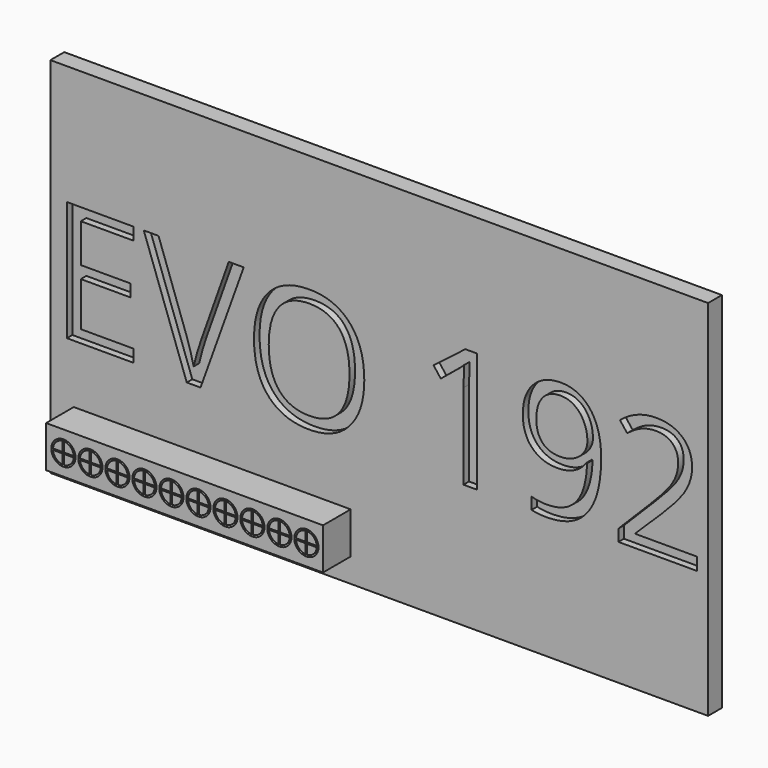
from build123d import *

# Parameters (mm, degrees)
F0_W         = 190
F0_H         = 105
F1_DEPTH     = 5
F2_TEXT_SIZE = 48.5157995531
F3_DEPTH     = 2
F4_W         = 80
F4_H         = 12
F4_R         = 3.5
F5_DEPTH     = 10


# Not quite as in the source:
# - Text() gives the source's letters only with a copy of the font that has no kerning and outlines rounded to 1/6400 em; it was checked with that copy


with BuildPart() as f1:
    # F0 (on Front) → F1 (new body)
    with BuildSketch(Plane.XZ):
        Rectangle(F0_W, F0_H)
    extrude(amount=F1_DEPTH)

    # F2 (on face) → F3 (cut)
    with BuildSketch(Plane.XZ.offset(5)):
        with Locations((-95, -16.6787064434)):
            Text('EVO 192', F2_TEXT_SIZE, font='Open Sans', text_align=(TextAlign.LEFT, TextAlign.BOTTOM))
    extrude(amount=-F3_DEPTH, mode=Mode.SUBTRACT)

    # F4 (on face) → F5 (join)
    with BuildSketch(Plane.XZ.offset(5)):
        with Locations((-48.2472097501, -39.5428631023)):
            Rectangle(F4_W, F4_H)
        with Locations((-83.2472097501, -39.5428631023)):
            Circle(F4_R, mode=Mode.SUBTRACT)
        with Locations((-75.4472097501, -39.5428631023)):
            Circle(F4_R, mode=Mode.SUBTRACT)
        with Locations((-67.6472097501, -39.5428631023)):
            Circle(F4_R, mode=Mode.SUBTRACT)
        with Locations((-59.8472097501, -39.5428631023)):
            Circle(F4_R, mode=Mode.SUBTRACT)
        with Locations((-52.0472097501, -39.5428631023)):
            Circle(F4_R, mode=Mode.SUBTRACT)
        with Locations((-44.2472097501, -39.5428631023)):
            Circle(F4_R, mode=Mode.SUBTRACT)
        with Locations((-36.4472097501, -39.5428631023)):
            Circle(F4_R, mode=Mode.SUBTRACT)
        with Locations((-28.6472097501, -39.5428631023)):
            Circle(F4_R, mode=Mode.SUBTRACT)
        with Locations((-20.8472097501, -39.5428631023)):
            Circle(F4_R, mode=Mode.SUBTRACT)
        with Locations((-13.0472097501, -39.5428631023)):
            Circle(F4_R, mode=Mode.SUBTRACT)
        with BuildLine():
            Line((-83.4472097501, -39.3428631023), (-83.4472097501, -36.5495371929))
            ThreePointArc((-83.4472097501, -36.5495371929), (-85.3685300937, -37.4215427588), (-86.2405356595, -39.3428631023))
            Line((-86.2405356595, -39.3428631023), (-83.4472097501, -39.3428631023))
        make_face()
        with BuildLine():
            Line((-83.0472097501, -39.3428631023), (-80.2538838407, -39.3428631023))
            ThreePointArc((-80.2538838407, -39.3428631023), (-81.1258894066, -37.4215427588), (-83.0472097501, -36.5495371929))
            Line((-83.0472097501, -36.5495371929), (-83.0472097501, -39.3428631023))
        make_face()
        with BuildLine():
            ThreePointArc((-83.0472097501, -42.5361890118), (-81.1258894066, -41.6641834459), (-80.2538838407, -39.7428631023))
            Line((-80.2538838407, -39.7428631023), (-83.0472097501, -39.7428631023))
            Line((-83.0472097501, -39.7428631023), (-83.0472097501, -42.5361890118))
        make_face()
        with BuildLine():
            ThreePointArc((-86.2405356595, -39.7428631023), (-85.3685300937, -41.6641834459), (-83.4472097501, -42.5361890118))
            Line((-83.4472097501, -42.5361890118), (-83.4472097501, -39.7428631023))
            Line((-83.4472097501, -39.7428631023), (-86.2405356595, -39.7428631023))
        make_face()
        with BuildLine():
            Line((-75.6472097501, -39.3428631023), (-75.6472097501, -36.5495371929))
            ThreePointArc((-75.6472097501, -36.5495371929), (-77.5685300937, -37.4215427588), (-78.4405356595, -39.3428631023))
            Line((-78.4405356595, -39.3428631023), (-75.6472097501, -39.3428631023))
        make_face()
        with BuildLine():
            Line((-75.2472097501, -39.3428631023), (-72.4538838407, -39.3428631023))
            ThreePointArc((-72.4538838407, -39.3428631023), (-73.3258894066, -37.4215427588), (-75.2472097501, -36.5495371929))
            Line((-75.2472097501, -36.5495371929), (-75.2472097501, -39.3428631023))
        make_face()
        with BuildLine():
            ThreePointArc((-75.2472097501, -42.5361890118), (-73.3258894066, -41.6641834459), (-72.4538838407, -39.7428631023))
            Line((-72.4538838407, -39.7428631023), (-75.2472097501, -39.7428631023))
            Line((-75.2472097501, -39.7428631023), (-75.2472097501, -42.5361890118))
        make_face()
        with BuildLine():
            ThreePointArc((-78.4405356595, -39.7428631023), (-77.5685300937, -41.6641834459), (-75.6472097501, -42.5361890118))
            Line((-75.6472097501, -42.5361890118), (-75.6472097501, -39.7428631023))
            Line((-75.6472097501, -39.7428631023), (-78.4405356595, -39.7428631023))
        make_face()
        with BuildLine():
            Line((-67.8472097501, -39.3428631023), (-67.8472097501, -36.5495371929))
            ThreePointArc((-67.8472097501, -36.5495371929), (-69.7685300937, -37.4215427588), (-70.6405356595, -39.3428631023))
            Line((-70.6405356595, -39.3428631023), (-67.8472097501, -39.3428631023))
        make_face()
        with BuildLine():
            Line((-67.4472097501, -39.3428631023), (-64.6538838407, -39.3428631023))
            ThreePointArc((-64.6538838407, -39.3428631023), (-65.5258894066, -37.4215427588), (-67.4472097501, -36.5495371929))
            Line((-67.4472097501, -36.5495371929), (-67.4472097501, -39.3428631023))
        make_face()
        with BuildLine():
            ThreePointArc((-67.4472097501, -42.5361890118), (-65.5258894066, -41.6641834459), (-64.6538838407, -39.7428631023))
            Line((-64.6538838407, -39.7428631023), (-67.4472097501, -39.7428631023))
            Line((-67.4472097501, -39.7428631023), (-67.4472097501, -42.5361890118))
        make_face()
        with BuildLine():
            ThreePointArc((-70.6405356595, -39.7428631023), (-69.7685300937, -41.6641834459), (-67.8472097501, -42.5361890118))
            Line((-67.8472097501, -42.5361890118), (-67.8472097501, -39.7428631023))
            Line((-67.8472097501, -39.7428631023), (-70.6405356595, -39.7428631023))
        make_face()
        with BuildLine():
            Line((-60.0472097501, -39.3428631023), (-60.0472097501, -36.5495371929))
            ThreePointArc((-60.0472097501, -36.5495371929), (-61.9685300937, -37.4215427588), (-62.8405356595, -39.3428631023))
            Line((-62.8405356595, -39.3428631023), (-60.0472097501, -39.3428631023))
        make_face()
        with BuildLine():
            Line((-59.6472097501, -39.3428631023), (-56.8538838407, -39.3428631023))
            ThreePointArc((-56.8538838407, -39.3428631023), (-57.7258894066, -37.4215427588), (-59.6472097501, -36.5495371929))
            Line((-59.6472097501, -36.5495371929), (-59.6472097501, -39.3428631023))
        make_face()
        with BuildLine():
            ThreePointArc((-59.6472097501, -42.5361890118), (-57.7258894066, -41.6641834459), (-56.8538838407, -39.7428631023))
            Line((-56.8538838407, -39.7428631023), (-59.6472097501, -39.7428631023))
            Line((-59.6472097501, -39.7428631023), (-59.6472097501, -42.5361890118))
        make_face()
        with BuildLine():
            ThreePointArc((-62.8405356595, -39.7428631023), (-61.9685300937, -41.6641834459), (-60.0472097501, -42.5361890118))
            Line((-60.0472097501, -42.5361890118), (-60.0472097501, -39.7428631023))
            Line((-60.0472097501, -39.7428631023), (-62.8405356595, -39.7428631023))
        make_face()
        with BuildLine():
            Line((-52.2472097501, -39.3428631023), (-52.2472097501, -36.5495371929))
            ThreePointArc((-52.2472097501, -36.5495371929), (-54.1685300937, -37.4215427588), (-55.0405356595, -39.3428631023))
            Line((-55.0405356595, -39.3428631023), (-52.2472097501, -39.3428631023))
        make_face()
        with BuildLine():
            Line((-51.8472097501, -39.3428631023), (-49.0538838407, -39.3428631023))
            ThreePointArc((-49.0538838407, -39.3428631023), (-49.9258894066, -37.4215427588), (-51.8472097501, -36.5495371929))
            Line((-51.8472097501, -36.5495371929), (-51.8472097501, -39.3428631023))
        make_face()
        with BuildLine():
            ThreePointArc((-51.8472097501, -42.5361890118), (-49.9258894066, -41.6641834459), (-49.0538838407, -39.7428631023))
            Line((-49.0538838407, -39.7428631023), (-51.8472097501, -39.7428631023))
            Line((-51.8472097501, -39.7428631023), (-51.8472097501, -42.5361890118))
        make_face()
        with BuildLine():
            ThreePointArc((-55.0405356595, -39.7428631023), (-54.1685300937, -41.6641834459), (-52.2472097501, -42.5361890118))
            Line((-52.2472097501, -42.5361890118), (-52.2472097501, -39.7428631023))
            Line((-52.2472097501, -39.7428631023), (-55.0405356595, -39.7428631023))
        make_face()
        with BuildLine():
            Line((-44.4472097501, -39.3428631023), (-44.4472097501, -36.5495371929))
            ThreePointArc((-44.4472097501, -36.5495371929), (-46.3685300937, -37.4215427588), (-47.2405356595, -39.3428631023))
            Line((-47.2405356595, -39.3428631023), (-44.4472097501, -39.3428631023))
        make_face()
        with BuildLine():
            Line((-44.0472097501, -39.3428631023), (-41.2538838407, -39.3428631023))
            ThreePointArc((-41.2538838407, -39.3428631023), (-42.1258894066, -37.4215427588), (-44.0472097501, -36.5495371929))
            Line((-44.0472097501, -36.5495371929), (-44.0472097501, -39.3428631023))
        make_face()
        with BuildLine():
            ThreePointArc((-44.0472097501, -42.5361890118), (-42.1258894066, -41.6641834459), (-41.2538838407, -39.7428631023))
            Line((-41.2538838407, -39.7428631023), (-44.0472097501, -39.7428631023))
            Line((-44.0472097501, -39.7428631023), (-44.0472097501, -42.5361890118))
        make_face()
        with BuildLine():
            ThreePointArc((-47.2405356595, -39.7428631023), (-46.3685300937, -41.6641834459), (-44.4472097501, -42.5361890118))
            Line((-44.4472097501, -42.5361890118), (-44.4472097501, -39.7428631023))
            Line((-44.4472097501, -39.7428631023), (-47.2405356595, -39.7428631023))
        make_face()
        with BuildLine():
            Line((-36.2472097501, -39.3428631023), (-33.4538838407, -39.3428631023))
            ThreePointArc((-33.4538838407, -39.3428631023), (-34.3258894066, -37.4215427588), (-36.2472097501, -36.5495371929))
            Line((-36.2472097501, -36.5495371929), (-36.2472097501, -39.3428631023))
        make_face()
        with BuildLine():
            Line((-36.6472097501, -39.3428631023), (-36.6472097501, -36.5495371929))
            ThreePointArc((-36.6472097501, -36.5495371929), (-38.5685300937, -37.4215427588), (-39.4405356595, -39.3428631023))
            Line((-39.4405356595, -39.3428631023), (-36.6472097501, -39.3428631023))
        make_face()
        with BuildLine():
            ThreePointArc((-39.4405356595, -39.7428631023), (-38.5685300937, -41.6641834459), (-36.6472097501, -42.5361890118))
            Line((-36.6472097501, -42.5361890118), (-36.6472097501, -39.7428631023))
            Line((-36.6472097501, -39.7428631023), (-39.4405356595, -39.7428631023))
        make_face()
        with BuildLine():
            ThreePointArc((-36.2472097501, -42.5361890118), (-34.3258894066, -41.6641834459), (-33.4538838407, -39.7428631023))
            Line((-33.4538838407, -39.7428631023), (-36.2472097501, -39.7428631023))
            Line((-36.2472097501, -39.7428631023), (-36.2472097501, -42.5361890118))
        make_face()
        with BuildLine():
            Line((-28.8472097501, -39.3428631023), (-28.8472097501, -36.5495371929))
            ThreePointArc((-28.8472097501, -36.5495371929), (-30.7685300937, -37.4215427588), (-31.6405356595, -39.3428631023))
            Line((-31.6405356595, -39.3428631023), (-28.8472097501, -39.3428631023))
        make_face()
        with BuildLine():
            Line((-28.4472097501, -39.3428631023), (-25.6538838407, -39.3428631023))
            ThreePointArc((-25.6538838407, -39.3428631023), (-26.5258894066, -37.4215427588), (-28.4472097501, -36.5495371929))
            Line((-28.4472097501, -36.5495371929), (-28.4472097501, -39.3428631023))
        make_face()
        with BuildLine():
            ThreePointArc((-28.4472097501, -42.5361890118), (-26.5258894066, -41.6641834459), (-25.6538838407, -39.7428631023))
            Line((-25.6538838407, -39.7428631023), (-28.4472097501, -39.7428631023))
            Line((-28.4472097501, -39.7428631023), (-28.4472097501, -42.5361890118))
        make_face()
        with BuildLine():
            ThreePointArc((-31.6405356595, -39.7428631023), (-30.7685300937, -41.6641834459), (-28.8472097501, -42.5361890118))
            Line((-28.8472097501, -42.5361890118), (-28.8472097501, -39.7428631023))
            Line((-28.8472097501, -39.7428631023), (-31.6405356595, -39.7428631023))
        make_face()
        with BuildLine():
            Line((-21.0472097501, -39.3428631023), (-21.0472097501, -36.5495371929))
            ThreePointArc((-21.0472097501, -36.5495371929), (-22.9685300937, -37.4215427588), (-23.8405356595, -39.3428631023))
            Line((-23.8405356595, -39.3428631023), (-21.0472097501, -39.3428631023))
        make_face()
        with BuildLine():
            Line((-20.6472097501, -39.3428631023), (-17.8538838407, -39.3428631023))
            ThreePointArc((-17.8538838407, -39.3428631023), (-18.7258894066, -37.4215427588), (-20.6472097501, -36.5495371929))
            Line((-20.6472097501, -36.5495371929), (-20.6472097501, -39.3428631023))
        make_face()
        with BuildLine():
            ThreePointArc((-20.6472097501, -42.5361890118), (-18.7258894066, -41.6641834459), (-17.8538838407, -39.7428631023))
            Line((-17.8538838407, -39.7428631023), (-20.6472097501, -39.7428631023))
            Line((-20.6472097501, -39.7428631023), (-20.6472097501, -42.5361890118))
        make_face()
        with BuildLine():
            ThreePointArc((-23.8405356595, -39.7428631023), (-22.9685300937, -41.6641834459), (-21.0472097501, -42.5361890118))
            Line((-21.0472097501, -42.5361890118), (-21.0472097501, -39.7428631023))
            Line((-21.0472097501, -39.7428631023), (-23.8405356595, -39.7428631023))
        make_face()
        with BuildLine():
            Line((-13.2472097501, -39.3428631023), (-13.2472097501, -36.5495371929))
            ThreePointArc((-13.2472097501, -36.5495371929), (-15.1685300937, -37.4215427588), (-16.0405356595, -39.3428631023))
            Line((-16.0405356595, -39.3428631023), (-13.2472097501, -39.3428631023))
        make_face()
        with BuildLine():
            Line((-12.8472097501, -39.3428631023), (-10.0538838407, -39.3428631023))
            ThreePointArc((-10.0538838407, -39.3428631023), (-10.9258894066, -37.4215427588), (-12.8472097501, -36.5495371929))
            Line((-12.8472097501, -36.5495371929), (-12.8472097501, -39.3428631023))
        make_face()
        with BuildLine():
            ThreePointArc((-12.8472097501, -42.5361890118), (-10.9258894066, -41.6641834459), (-10.0538838407, -39.7428631023))
            Line((-10.0538838407, -39.7428631023), (-12.8472097501, -39.7428631023))
            Line((-12.8472097501, -39.7428631023), (-12.8472097501, -42.5361890118))
        make_face()
        with BuildLine():
            ThreePointArc((-16.0405356595, -39.7428631023), (-15.1685300937, -41.6641834459), (-13.2472097501, -42.5361890118))
            Line((-13.2472097501, -42.5361890118), (-13.2472097501, -39.7428631023))
            Line((-13.2472097501, -39.7428631023), (-16.0405356595, -39.7428631023))
        make_face()
    extrude(amount=F5_DEPTH)


solid = f1.part
